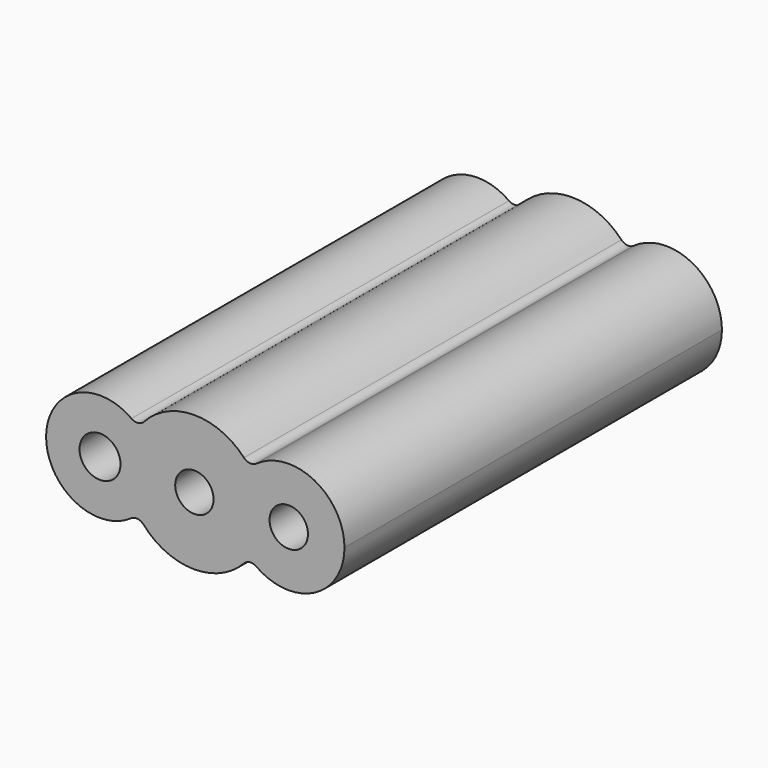
from build123d import *

# Parameters (mm, degrees)
F1_DEPTH = 254
F2_R     = 5.08
F3_R     = 11.0334695749
F3_R_2   = 10.3236193182
F3_R_3   = 10.3446634655
F4_DEPTH = 461.264


# Not quite as in the source:
# - the program builds the solid bodies; features that only make, move or delete a surface that nothing else refers to are left out


with BuildPart() as f1:
    # F0 (on Front) → F1 (new body)
    with BuildSketch(Plane.XZ):
        with BuildLine():
            ThreePointArc((-30.4000387615, -20.3651585358), (-24.0059784619, -10.8970905515), (-21.758691331, 0.3046065976))
            ThreePointArc((-21.758691331, 0.3046065976), (-23.9392938004, 11.3454431448), (-30.1536347581, 20.7282500411))
            ThreePointArc((-30.1536347581, 20.7282500411), (-36.5903525714, 0.2194028111), (-30.4000387615, -20.3651585358))
        make_face()
        with BuildLine():
            ThreePointArc((-30.1536347581, 20.7282500411), (-23.9392938004, 11.3454431448), (-21.758691331, 0.3046065976))
            ThreePointArc((-21.758691331, 0.3046065976), (-24.0059784619, -10.8970905515), (-30.4000387615, -20.3651585358))
            ThreePointArc((-30.4000387615, -20.3651585358), (-0.593995823, -36.5861887582), (29.7229129207, -21.3412859593))
            ThreePointArc((29.7229129207, -21.3412859593), (20.8050989976, 0), (29.7229129207, 21.3412859593))
            ThreePointArc((29.7229129207, 21.3412859593), (-0.3746112446, 36.5890927095), (-30.1536347581, 20.7282500411))
        make_face()
        with BuildLine():
            ThreePointArc((-30.4000387615, -20.3651585358), (-36.5903525714, 0.2194028111), (-30.1536347581, 20.7282500411))
            ThreePointArc((-30.1536347581, 20.7282500411), (-79.8407866027, 0.4787407551), (-30.4000387615, -20.3651585358))
        make_face()
        with BuildLine():
            ThreePointArc((36.5910103562, 0), (34.8316914131, 11.2096080304), (29.7229129207, 21.3412859593))
            ThreePointArc((29.7229129207, 21.3412859593), (20.8050989976, 0), (29.7229129207, -21.3412859593))
            ThreePointArc((29.7229129207, -21.3412859593), (34.8316914131, -11.2096080304), (36.5910103562, 0))
        make_face()
        with BuildLine():
            ThreePointArc((80.7949010024, 0), (62.364794546, 27.6757947177), (29.7229129207, 21.3412859593))
            ThreePointArc((29.7229129207, 21.3412859593), (34.8316914131, 11.2096080304), (36.5910103562, 0))
            ThreePointArc((36.5910103562, 0), (34.8316914131, -11.2096080304), (29.7229129207, -21.3412859593))
            ThreePointArc((29.7229129207, -21.3412859593), (62.364794546, -27.6757947177), (80.7949010024, 0))
        make_face()
    extrude(amount=F1_DEPTH)

    # F2
    f2_edges = [f1.edges().sort_by_distance(p)[0] for p in [
        (29.722913, -127, 21.341286),
        (-30.153635, -127, 20.72825),
        (29.722913, -127, -21.341286),
        (-30.400039, -127, -20.365159),
    ]]
    fillet(f2_edges, radius=F2_R)

    # F3 (on face) → F4 (cut)
    with BuildSketch(Plane.XZ.offset(254)):
        with Locations((-50.8, 0.3046065976)):
            Circle(F3_R)
        Circle(F3_R_2)
        with Locations((50.8, 0)):
            Circle(F3_R_3)
    extrude(amount=-F4_DEPTH, mode=Mode.SUBTRACT)


solid = f1.part
